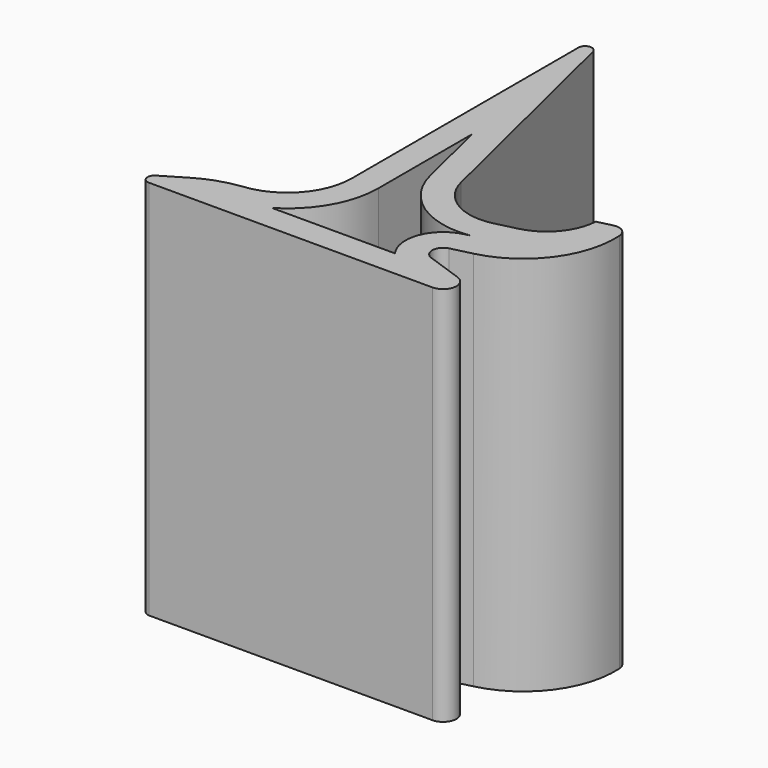
from build123d import *

# Parameters (mm, degrees)
F1_DEPTH     = 76.2
F2_DEPTH     = 15.24
F3_R         = 12.8774151417
F4_R         = 20.6186868219
F5_T1_DEPTH  = 101.180790156
F6_R         = 2.2113922374
F7_T1_DEPTH  = 154.3936506005
F8_T1_DEPTH  = 132.0243451665
F9_T1_DEPTH  = 76.2
F10_T1_DEPTH = 168.1440052245
F11_R        = 2.3364132001
F12_T        = -5.334


# Not quite as in the source:
# - a fillet or chamfer that OpenCascade refuses, or shapes differently, is made with other operations: its cross-section is extruded or revolved along the edge and cut away or added


with BuildPart() as f1:
    # F0 (on Top) → F1 (new body)
    with BuildSketch(Plane.XY):
        Polygon((-23.9872187376, -31.7199416459), (-47.0275729895, 62.9664510489), (-55.8593086898, 62.9664510489), (-55.8593086898, -44.0704375505), (-69.4310441613, -52.1240867674), (7.9028792679, -52.1240867674), (-21.2087563334, -41.9485626592), (8.002824487, -34.8404117285), (3.777547454, -17.4762585554), (-1.7201294546, -18.8140265274), (0, -25.8830520834), align=None)
    extrude(amount=F1_DEPTH)

    # F2 (cut): a face of the model
    f2_faces = [f1.faces().sort_by_distance(p)[0] for p in [
        (-55.8593086898, 9.4480067492, 38.1),
    ]]
    extrude(f2_faces, amount=-F2_DEPTH, mode=Mode.SUBTRACT)

    # F3
    f3_edges = [f1.edges().sort_by_distance(p)[0] for p in [
        (-40.619309, -44.070438, 38.1),
    ]]
    fillet(f3_edges, radius=F3_R)

    # F4
    f4_edges = [f1.edges().sort_by_distance(p)[0] for p in [
        (-55.859309, -44.070438, 38.1),
    ]]
    fillet(f4_edges, radius=F4_R)

    # F5: fillet of radius 1.3707998783 on 1 edges, made by hand

    # F5_s2 → F5_t1 (cut)
    with BuildSketch(Plane.XY.offset(-12.490395078)):
        with BuildLine():
            ThreePointArc((-65.1344391621, -49.5744239362), (-65.7568311931, -51.1159900142), (-64.4348861301, -52.1240867674))
            Line((-64.4348861301, -52.1240867674), (-69.4310441613, -52.1240867674))
            Line((-69.4310441613, -52.1240867674), (-65.1344391621, -49.5744239362))
        make_face()
    extrude(amount=F5_T1_DEPTH, mode=Mode.SUBTRACT)

    # F6
    f6_edges = [f1.edges().sort_by_distance(p)[0] for p in [
        (-21.208756, -41.948563, 38.1),
    ]]
    fillet(f6_edges, radius=F6_R)

    # F7: fillet of radius 2.6543994462 on 1 edges, made by hand

    # F7_s2 → F7_t1 (cut)
    with BuildSketch(Plane.XY.offset(-39.0968253003)):
        with BuildLine():
            ThreePointArc((-6.8600078332, -46.9639468268), (-5.1188800269, -49.913872102), (-7.7358508522, -52.1240867674))
            Line((-7.7358508522, -52.1240867674), (7.9028792679, -52.1240867674))
            Line((7.9028792679, -52.1240867674), (-6.8600078332, -46.9639468268))
        make_face()
    extrude(amount=F7_T1_DEPTH, mode=Mode.SUBTRACT)

    # F8: fillet of radius 1.3388584964 on 1 edges, made by hand

    # F8_s2 → F8_t1 (cut)
    with BuildSketch(Plane.XY.offset(-27.9121725832)):
        with BuildLine():
            ThreePointArc((-40.6193086898, 25.466247787), (-39.4398601206, 26.7955824133), (-37.979551683, 25.78279974))
            Line((-37.979551683, 25.78279974), (-40.6193086898, 36.6311168203))
            Line((-40.6193086898, 36.6311168203), (-40.6193086898, 25.466247787))
        make_face()
    extrude(amount=F8_T1_DEPTH, mode=Mode.SUBTRACT)

    # F9: fillet of radius 10.4245741623 on 2 edges, made by hand

    # F9_s2 → F9_t1 (join)
    with BuildSketch(Plane.XY):
        with BuildLine():
            ThreePointArc((-26.4519447103, -21.5909302259), (-21.7424015031, -28.031321364), (-13.8582073177, -29.2552156732))
            Line((-13.8582073177, -29.2552156732), (-23.9872187376, -31.7199416459))
            Line((-23.9872187376, -31.7199416459), (-26.4519447103, -21.5909302259))
        make_face()
        with BuildLine():
            ThreePointArc((-9.6557422738, -28.2326159037), (-4.1483336949, -24.8205098096), (-1.7201294546, -18.8140265274))
            Line((-1.7201294546, -18.8140265274), (0, -25.8830520834))
            Line((0, -25.8830520834), (-9.6557422738, -28.2326159037))
        make_face()
    extrude(amount=F9_T1_DEPTH)

    # F10: fillet of radius 18.3963073453 on 1 edges, made by hand

    # F10_s2 → F10_t1 (cut)
    with BuildSketch(Plane.XY.offset(-45.9720026122)):
        with BuildLine():
            ThreePointArc((3.777547454, -17.4762585554), (1.3625814789, -31.1006820929), (-9.8646080702, -39.1881534047))
            Line((-9.8646080702, -39.1881534047), (8.002824487, -34.8404117285))
            Line((8.002824487, -34.8404117285), (3.777547454, -17.4762585554))
        make_face()
    extrude(amount=F10_T1_DEPTH, mode=Mode.SUBTRACT)

    # F11
    f11_edges = [f1.edges().sort_by_distance(p)[0] for p in [
        (3.777547, -17.476259, 38.1),
    ]]
    fillet(f11_edges, radius=F11_R)

    # F12
    f12_openings = [f1.faces().sort_by_distance(p)[0] for p in [
        (-29.256427, -29.797459, 76.2),
        (-29.256427, -29.797459, 0),
    ]]
    offset(amount=F12_T, openings=f12_openings)


solid = f1.part
